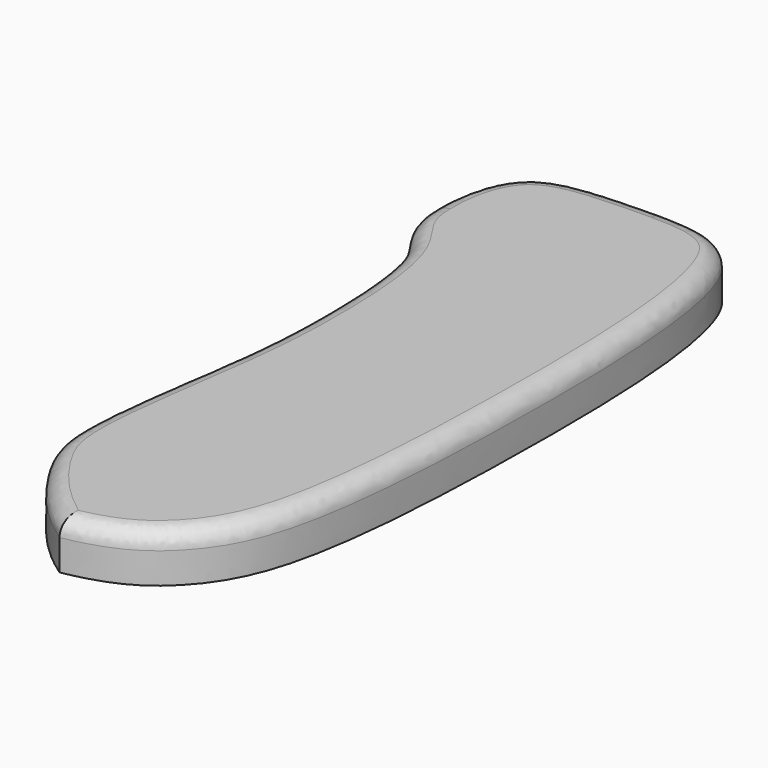
from build123d import *

# Parameters (mm, degrees)
F1_DEPTH = 8.73125
F2_R     = 3.175
F3_W     = 28.575
F3_H     = 127
F4_DEPTH = 6.35


with BuildPart() as f1:
    # F0 (on Top) → F1 (new body)
    with BuildSketch(Plane.XY):
        with BuildLine():
            add(Edge.make_bspline(
                [(-22.2630089622, 57.15), (-22.4771988152, 63.2990440352), (-19.5114240111, 73.9089506041), (-6.4019025255, 76.1693999245), (1.1398358038, 76.1729106307), (4.6904176342, 76.2)],
                knots=[0, 0, 0, 0, 0.3691493182, 0.6877576776, 1, 1, 1, 1], degree=3))
            add(Edge.make_bspline(
                [(-22.2630089622, 57.15), (-22.2630089622, 50.8514460964), (-15.3473480842, 46.9394491864), (-13.8715606343, 22.3627512215), (-15.0570255507, 3.0651518011), (-20.4466410587, -27.8145738651), (-16.0074621044, -38.1660419017), (-9.4359992072, -46.521846205), (-3.2130089622, -50.7988970175)],
                knots=[0, 0, 0, 0, 0.138868117, 0.3185437234, 0.4995856975, 0.7107090098, 0.8363339586, 1, 1, 1, 1], degree=3))
            add(Edge.make_bspline(
                [(4.6904176342, 76.2), (14.5339909941, 76.3216987252), (24.2244258774, 70.1525650219), (25.3902250152, 16.8633127605), (22.7411357456, -28.7061581774), (13.1823598211, -43.9861209726), (5.1097106189, -49.3051670492), (-3.2130089622, -50.7988970175)],
                knots=[0, 0, 0, 0, 0.1602601979, 0.4302268246, 0.6912927459, 0.8402816289, 1, 1, 1, 1], degree=3))
        make_face()
    extrude(amount=F1_DEPTH)

    # F2
    f2_edges = [f1.edges().sort_by_distance(p)[0] for p in [
        (-14.65314, 73.993268, 8.73125),
        (24.530161, 12.135146, 8.73125),
        (-15.806546, 1.03866, 8.73125),
    ]]
    fillet(f2_edges, radius=F2_R)

    # F3 (on face) → F4 (cut)
    with BuildSketch(Plane(origin=(0, 0, 0), x_dir=(1, 0, 0), z_dir=(0, 0, -1))):
        with Locations((3.1477137653, -38.1)):
            Rectangle(F3_W, F3_H)
    extrude(amount=-F4_DEPTH, mode=Mode.SUBTRACT)


solid = f1.part
